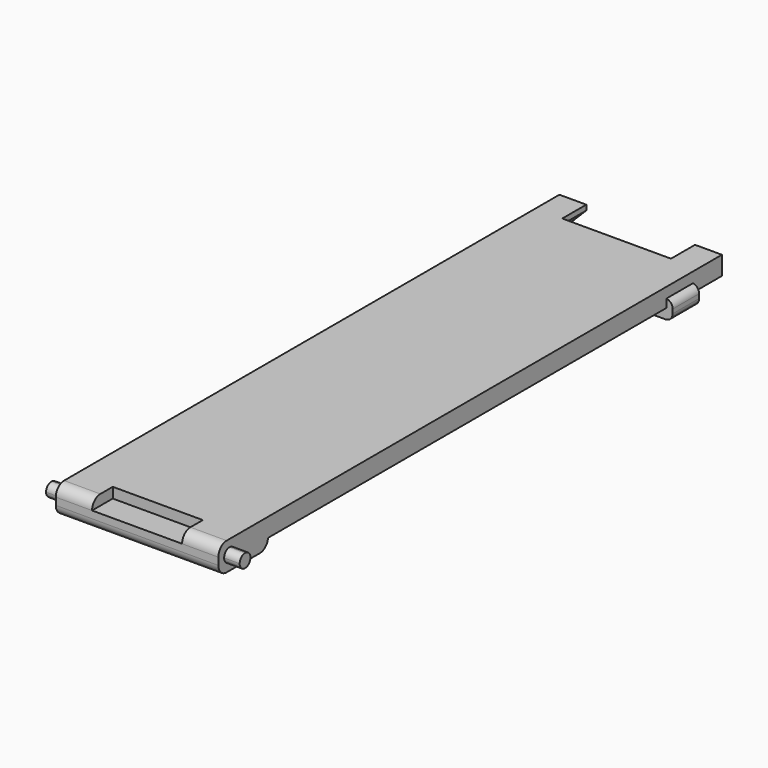
from build123d import *

# Parameters (mm, degrees)
F0_W         = 2.3
F0_H         = 3.2
F1_DEPTH     = 1.8
F0_W_2       = 8.7
F0_H_2       = 2.5
F2_DEPTH     = 0.9
F0_W_3       = 0.6
F3_DEPTH     = 1
F4_DEPTH     = 0.8
F5_DEPTH     = 0.8
F6_T4_DEPTH  = 9.5863757687
F6_T10_DEPTH = 9.5863757687
F6_T16_DEPTH = 17.1863757687
F6_T23_DEPTH = 17.1863757687
F6_T31_DEPTH = 9.5863757687
F6_T37_DEPTH = 9.5863757687
F7_T1_DEPTH  = 6.6641016151
F7_T3_DEPTH  = 6.7
F8_T1_DEPTH  = 8.5
F8_T3_DEPTH  = 20.7
F8_T5_DEPTH  = 8.5
F8_T7_DEPTH  = 20.6749371855
F0_W_4       = 1.5
F0_H_3       = 1.3
F9_DEPTH     = 0.2
F10_DEPTH    = 1.1
F11_R        = 0.64999
F12_R        = 0.64999


# Not quite as in the source:
# - a fillet or chamfer that OpenCascade refuses, or shapes differently, is made with other operations: its cross-section is extruded or revolved along the edge and cut away or added
# - a fillet or chamfer is up to 0.001 mm smaller than in the source, because OpenCascade refuses the exact size


with BuildPart() as f1:
    # F0 (on Top) → F1 (new body)
    with BuildSketch(Plane.XY):
        Polygon((8.8998297817, -13.0360927206), (-6.8001702183, -13.0360927206), (-6.8001702183, -16.0360927206), (-6.8001702183, -17.0360927206), (-6.8001702183, -18.3360927206), (-6.8001702183, -19.0360927206), (-3.3001702183, -19.0360927206), (-3.3001702183, -16.5360927206), (5.3998297817, -16.5360927206), (5.3998297817, -19.0360927206), (8.8998297817, -19.0360927206), (8.8998297817, -18.3360927206), (8.8998297817, -17.0360927206), align=None)
        Polygon((-4.2001702183, 41.7639072794), (-6.8001702183, 41.7639072794), (-6.8001702183, 38.2639072794), (-4.5001702183, 38.2639072794), (-4.5001702183, 35.0639072794), (-6.8001702183, 35.0639072794), (-6.8001702183, -13.0360927206), (8.8998297817, -13.0360927206), (8.8998297817, 35.0639072794), (6.5998297817, 35.0639072794), (6.5998297817, 38.2639072794), (8.8998297817, 38.2639072794), (8.8998297817, 41.7639072794), (6.2998297817, 41.7639072794), (6.2998297817, 38.8639072794), (-4.2001702183, 38.8639072794), align=None)
        with Locations((7.7498297817, 36.6639072794)):
            Rectangle(F0_W, F0_H)
        with Locations((-5.6501702183, 36.6639072794)):
            Rectangle(F0_W, F0_H)
    extrude(amount=F1_DEPTH)

    # F0 (on Top) → F2 (join)
    with BuildSketch(Plane.XY):
        with Locations((1.0498297817, -17.7860927206)):
            Rectangle(F0_W_2, F0_H_2)
        Polygon((8.8998297817, -13.0360927206), (-6.8001702183, -13.0360927206), (-6.8001702183, -16.0360927206), (-6.8001702183, -17.0360927206), (-6.8001702183, -18.3360927206), (-6.8001702183, -19.0360927206), (-3.3001702183, -19.0360927206), (-3.3001702183, -16.5360927206), (5.3998297817, -16.5360927206), (5.3998297817, -19.0360927206), (8.8998297817, -19.0360927206), (8.8998297817, -18.3360927206), (8.8998297817, -17.0360927206), align=None)
    extrude(amount=-F2_DEPTH)

    # F0 (on Top) → F3 (join)
    with BuildSketch(Plane.XY):
        with Locations((7.7498297817, 36.6639072794)):
            Rectangle(F0_W, F0_H)
        with Locations((9.1998297817, 36.6639072794)):
            Rectangle(F0_W_3, F0_H)
        with Locations((-5.6501702183, 36.6639072794)):
            Rectangle(F0_W, F0_H)
        with Locations((-7.1001702183, 36.6639072794)):
            Rectangle(F0_W_3, F0_H)
    extrude(amount=-F3_DEPTH)

    # F0 (on Top) → F4 (join)
    with BuildSketch(Plane.XY):
        with Locations((9.1998297817, 36.6639072794)):
            Rectangle(F0_W_3, F0_H)
        with Locations((-7.1001702183, 36.6639072794)):
            Rectangle(F0_W_3, F0_H)
    extrude(amount=F4_DEPTH)

    # F0 (on Top) → F5 (join)
    with BuildSketch(Plane.XY):
        with Locations((1.0498297817, -17.7860927206)):
            Rectangle(F0_W_2, F0_H_2)
    extrude(amount=F5_DEPTH)

    # F6: chamfer of 1.3 on 3 edges, made by hand


with BuildPart() as f6_tool2:
    # F6_s3 → F6_t4 (new body)
    with BuildSketch(Plane.XZ.offset(-45.1070951637)):
        Polygon((7.5998297817, 0), (6.2998297817, 1.3), (6.2998297817, 0), align=None)
    extrude(amount=F6_T4_DEPTH)

    split(bisect_by=Plane.XZ.offset(-38.2639072794), keep=Keep.BOTTOM)

    split(bisect_by=Plane(origin=(0, 18.7819536397, -18.7819536397), x_dir=(1, 0, 0), z_dir=(0, 0.7071067812, -0.7071067812)), keep=Keep.TOP)


with BuildPart() as f1_1:
    add(f1.part)

    # F6_t1: cut F6_tool2
    add(f6_tool2.part, mode=Mode.SUBTRACT)


with BuildPart() as f6_tool8:
    # F6_s9 → F6_t10 (new body)
    with BuildSketch(Plane.XZ.offset(-45.1070951637)):
        Polygon((7.5998297817, 0), (6.2998297817, 1.3), (6.2998297817, 0), align=None)
    extrude(amount=F6_T10_DEPTH)

    split(bisect_by=Plane.YZ.offset(6.5998297817), keep=Keep.BOTTOM)

    split(bisect_by=Plane(origin=(0, 18.7819536397, -18.7819536397), x_dir=(1, 0, 0), z_dir=(0, 0.7071067812, -0.7071067812)), keep=Keep.TOP)


with BuildPart() as f1_2:
    add(f1_1.part)

    # F6_t7: cut F6_tool8
    add(f6_tool8.part, mode=Mode.SUBTRACT)


with BuildPart() as f6_tool14:
    # F6_s15 → F6_t16 (new body)
    with BuildSketch(Plane.YZ.offset(9.6430176661)):
        Polygon((37.5639072794, 0), (38.8639072794, 1.3), (38.8639072794, 0), align=None)
    extrude(amount=-F6_T16_DEPTH)

    split(bisect_by=Plane.XZ.offset(-38.2639072794), keep=Keep.BOTTOM)

    split(bisect_by=Plane(origin=(-2.7500851092, 0, 2.7500851092), x_dir=(0, 1, 0), z_dir=(0.7071067812, 0, -0.7071067812)), keep=Keep.TOP)

    split(bisect_by=Plane(origin=(3.7999148908, 0, 3.7999148908), x_dir=(0, 1, 0), z_dir=(-0.7071067812, 0, -0.7071067812)), keep=Keep.TOP)


with BuildPart() as f1_3:
    add(f1_2.part)

    # F6_t13: cut F6_tool14
    add(f6_tool14.part, mode=Mode.SUBTRACT)


with BuildPart() as f6_tool21:
    # F6_s22 → F6_t23 (new body)
    with BuildSketch(Plane.YZ.offset(9.6430176661)):
        Polygon((37.5639072794, 0), (38.8639072794, 1.3), (38.8639072794, 0), align=None)
    extrude(amount=-F6_T23_DEPTH)

    split(bisect_by=Plane.YZ.offset(6.5998297817), keep=Keep.BOTTOM)

    split(bisect_by=Plane.YZ.offset(-4.5001702183), keep=Keep.TOP)

    split(bisect_by=Plane(origin=(-2.7500851092, 0, 2.7500851092), x_dir=(0, 1, 0), z_dir=(0.7071067812, 0, -0.7071067812)), keep=Keep.TOP)

    split(bisect_by=Plane(origin=(3.7999148908, 0, 3.7999148908), x_dir=(0, 1, 0), z_dir=(-0.7071067812, 0, -0.7071067812)), keep=Keep.TOP)


with BuildPart() as f1_4:
    add(f1_3.part)

    # F6_t20: cut F6_tool21
    add(f6_tool21.part, mode=Mode.SUBTRACT)


with BuildPart() as f6_tool29:
    # F6_s30 → F6_t31 (new body)
    with BuildSketch(Plane.XZ.offset(-35.520719395)):
        Polygon((-5.5001702183, 0), (-4.2001702183, 1.3), (-4.2001702183, 0), align=None)
    extrude(amount=-F6_T31_DEPTH)

    split(bisect_by=Plane.YZ.offset(-4.5001702183), keep=Keep.TOP)

    split(bisect_by=Plane(origin=(0, 18.7819536397, -18.7819536397), x_dir=(1, 0, 0), z_dir=(0, 0.7071067812, -0.7071067812)), keep=Keep.TOP)


with BuildPart() as f1_5:
    add(f1_4.part)

    # F6_t28: cut F6_tool29
    add(f6_tool29.part, mode=Mode.SUBTRACT)


with BuildPart() as f6_tool35:
    # F6_s36 → F6_t37 (new body)
    with BuildSketch(Plane.XZ.offset(-35.520719395)):
        Polygon((-5.5001702183, 0), (-4.2001702183, 1.3), (-4.2001702183, 0), align=None)
    extrude(amount=-F6_T37_DEPTH)

    split(bisect_by=Plane.XZ.offset(-38.2639072794), keep=Keep.BOTTOM)

    split(bisect_by=Plane(origin=(0, 18.7819536397, -18.7819536397), x_dir=(1, 0, 0), z_dir=(0, 0.7071067812, -0.7071067812)), keep=Keep.TOP)


with BuildPart() as f1_6:
    add(f1_5.part)

    # F6_t34: cut F6_tool35
    add(f6_tool35.part, mode=Mode.SUBTRACT)

    # F7: fillet of radius 0.7 on 6 edges, made by hand

    # F7_s2 → F7_t1 (cut)
    with BuildSketch(Plane.XZ.offset(-39.9959580869)):
        with BuildLine():
            ThreePointArc((-7.4001702183, 0.107179677), (-7.2293204805, 0.5654372465), (-6.8001702183, 0.8))
            Line((-6.8001702183, 0.8), (-7.4001702183, 0.8))
            Line((-7.4001702183, 0.8), (-7.4001702183, 0.107179677))
        make_face()
        with BuildLine():
            ThreePointArc((9.4998297817, 0.107179677), (9.3289800439, 0.5654372465), (8.8998297817, 0.8))
            Line((8.8998297817, 0.8), (9.4998297817, 0.8))
            Line((9.4998297817, 0.8), (9.4998297817, 0.107179677))
        make_face()
    extrude(amount=F7_T1_DEPTH, mode=Mode.SUBTRACT)

    # F7_s4 → F7_t3 (cut)
    with BuildSketch(Plane.XZ.offset(-40.0139072794)):
        with BuildLine():
            ThreePointArc((-6.7001702183, -1), (-7.1951449651, -0.7949747468), (-7.4001702183, -0.3))
            Line((-7.4001702183, -0.3), (-7.4001702183, -1))
            Line((-7.4001702183, -1), (-6.7001702183, -1))
        make_face()
        with BuildLine():
            ThreePointArc((-5.2001702183, -1), (-4.7051954715, -0.7949747468), (-4.5001702183, -0.3))
            Line((-4.5001702183, -0.3), (-4.5001702183, -1))
            Line((-4.5001702183, -1), (-5.2001702183, -1))
        make_face()
        with BuildLine():
            ThreePointArc((6.5998297817, -0.3), (6.8048550349, -0.7949747468), (7.2998297817, -1))
            Line((7.2998297817, -1), (6.5998297817, -1))
            Line((6.5998297817, -1), (6.5998297817, -0.3))
        make_face()
        with BuildLine():
            ThreePointArc((8.7998297817, -1), (9.2948045285, -0.7949747468), (9.4998297817, -0.3))
            Line((9.4998297817, -0.3), (9.4998297817, -1))
            Line((9.4998297817, -1), (8.7998297817, -1))
        make_face()
    extrude(amount=F7_T3_DEPTH, mode=Mode.SUBTRACT)

    # F8: fillet of radius 1 on 4 edges, made by hand

    # F8_s2 → F8_t1 (cut)
    with BuildSketch(Plane.YZ.offset(-9.3001702183)):
        with BuildLine():
            ThreePointArc((-19.0360927206, 0.8), (-18.7431995018, 1.5071067812), (-18.0360927206, 1.8))
            Line((-18.0360927206, 1.8), (-19.0360927206, 1.8))
            Line((-19.0360927206, 1.8), (-19.0360927206, 0.8))
        make_face()
    extrude(amount=F8_T1_DEPTH, mode=Mode.SUBTRACT)

    # F8_s4 → F8_t3 (cut)
    with BuildSketch(Plane.YZ.offset(-9.3001702183)):
        with BuildLine():
            ThreePointArc((-19.0360927206, 0.1), (-18.7431995018, -0.6071067812), (-18.0360927206, -0.9))
            Line((-18.0360927206, -0.9), (-19.0360927206, -0.9))
            Line((-19.0360927206, -0.9), (-19.0360927206, 0.1))
        make_face()
    extrude(amount=F8_T3_DEPTH, mode=Mode.SUBTRACT)

    # F8_s6 → F8_t5 (cut)
    with BuildSketch(Plane.YZ.offset(2.8998297817)):
        with BuildLine():
            ThreePointArc((-19.0360927206, 0.8), (-18.7431995018, 1.5071067812), (-18.0360927206, 1.8))
            Line((-18.0360927206, 1.8), (-19.0360927206, 1.8))
            Line((-19.0360927206, 1.8), (-19.0360927206, 0.8))
        make_face()
    extrude(amount=F8_T5_DEPTH, mode=Mode.SUBTRACT)

    # F8_s8 → F8_t7 (cut)
    with BuildSketch(Plane.YZ.offset(-9.2876388111)):
        with BuildLine():
            ThreePointArc((-14.0310801578, -0.9), (-13.3602597645, -0.6416198487), (-13.0360927206, 0))
            Line((-13.0360927206, 0), (-13.0360927206, -0.9))
            Line((-13.0360927206, -0.9), (-14.0310801578, -0.9))
        make_face()
    extrude(amount=F8_T7_DEPTH, mode=Mode.SUBTRACT)

    # F0 (on Top) → F9 (join)
    with BuildSketch(Plane.XY):
        with Locations((-7.5501702183, -17.6860927206)):
            Rectangle(F0_W_4, F0_H_3)
        with Locations((9.6498297817, -17.6860927206)):
            Rectangle(F0_W_4, F0_H_3)
    extrude(amount=-F9_DEPTH)

    # F0 (on Top) → F10 (join)
    with BuildSketch(Plane.XY):
        with Locations((-7.5501702183, -17.6860927206)):
            Rectangle(F0_W_4, F0_H_3)
        with Locations((9.6498297817, -17.6860927206)):
            Rectangle(F0_W_4, F0_H_3)
    extrude(amount=F10_DEPTH)

    # F11 (radius 0.65 in the source; OpenCascade refuses exactly that, so slightly less here)
    f11_edges = [f1_6.edges().sort_by_distance(p)[0] for p in [
        (9.64983, -17.036093, 1.1),
        (9.64983, -18.336093, 1.1),
    ]]
    fillet(f11_edges, radius=F11_R)

    # F12 (radius 0.65 in the source; OpenCascade refuses exactly that, so slightly less here)
    f12_edges = [f1_6.edges().sort_by_distance(p)[0] for p in [
        (9.64983, -18.336093, -0.2),
        (9.64983, -17.036093, -0.2),
        (-7.55017, -18.336093, -0.2),
        (-7.55017, -17.036093, -0.2),
        (-7.55017, -18.336093, 1.1),
        (-7.55017, -17.036093, 1.1),
    ]]
    fillet(f12_edges, radius=F12_R)


solid = f1_6.part
